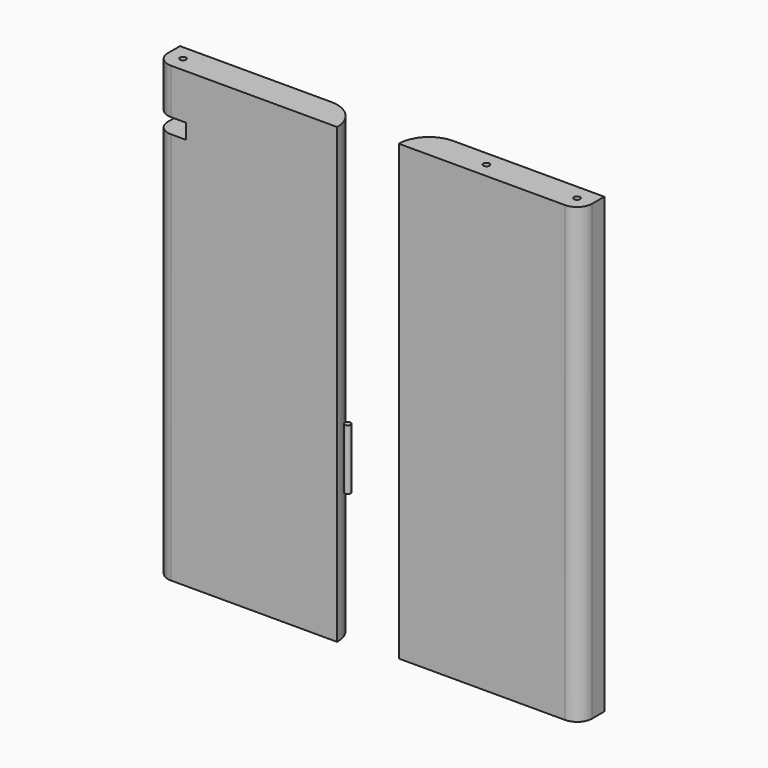
from build123d import *

# Parameters (mm, degrees)
F1_DEPTH  = 10
F0_W      = 60
F0_H      = 150
F2_R      = 5
F2_2_R    = 5
F4_R      = 9.99999
F4_2_R    = 9.99999
F3_W      = 30
F3_H      = 2
F5_DEPTH  = 8
F6_R      = 1
F7_DEPTH  = 20
F8_R      = 1
F9_DEPTH  = 10
F10_R     = 1
F11_DEPTH = 10
F12_R     = 1
F13_DEPTH = 10
F14_R     = 1
F15_DEPTH = 10
F16_R     = 1
F17_DEPTH = 20


# Not quite as in the source:
# - a fillet or chamfer is up to 0.001 mm smaller than in the source, because OpenCascade refuses the exact size


with BuildPart() as f1:
    # F0 (on Front) → F1 (new body)
    with BuildSketch(Plane.XZ):
        Polygon((-17.6528605427, 79.6767238528), (-77.6528605427, 79.6767238528), (-77.6528605427, 64.6767238528), (-67.6528605427, 64.6767238528), (-67.6528605427, 59.6767238528), (-77.6528605427, 59.6767238528), (-77.6528605427, -70.3232761472), (-17.6528605427, -70.3232761472), align=None)
    extrude(amount=F1_DEPTH)

    # F2
    f2_edges = [f1.edges().sort_by_distance(p)[0] for p in [
        (-77.652861, -10, 72.176724),
        (-77.652861, -10, -5.323276),
    ]]
    fillet(f2_edges, radius=F2_R)

    # F4#2 (radius 10 in the source; OpenCascade refuses exactly that, so slightly less here)
    f4_2_edges = [f1.edges().sort_by_distance(p)[0] for p in [
        (-17.652861, 0, 4.676724),
    ]]
    fillet(f4_2_edges, radius=F4_2_R)

    # F8 (on face) → F9 (cut)
    with BuildSketch(Plane(origin=(0, 0, -70.3232761472), x_dir=(1, 0, 0), z_dir=(0, 0, -1))):
        with Locations((-72.6528605427, 5)):
            Circle(F8_R)
    extrude(amount=-F9_DEPTH, mode=Mode.SUBTRACT)

    # F12 (on face) → F13 (cut)
    with BuildSketch(Plane.XY.offset(79.6767238528)):
        with Locations((-72.6528605427, -5)):
            Circle(F12_R)
    extrude(amount=-F13_DEPTH, mode=Mode.SUBTRACT)


with BuildPart() as f1b:
    # F0 (on Front) → F1, piece 2 (new body)
    with BuildSketch(Plane.XZ):
        with Locations((32.7451354545, 6.4557090402)):
            Rectangle(F0_W, F0_H)
    extrude(amount=F1_DEPTH)

    # F2#2
    f2_2_edges = [f1b.edges().sort_by_distance(p)[0] for p in [
        (62.745135, -10, 6.455709),
    ]]
    fillet(f2_2_edges, radius=F2_2_R)

    # F4 (radius 10 in the source; OpenCascade refuses exactly that, so slightly less here)
    f4_edges = [f1b.edges().sort_by_distance(p)[0] for p in [
        (2.745135, 0, 6.455709),
    ]]
    fillet(f4_edges, radius=F4_R)

    # F3 (on face) → F5 (cut)
    with BuildSketch(Plane(origin=(0, 0, 0), x_dir=(-1, 0, 0), z_dir=(0, 1, 0))):
        with Locations((-27.7451354545, 67.4557090402)):
            Rectangle(F3_W, F3_H)
    extrude(amount=-F5_DEPTH, mode=Mode.SUBTRACT)

    # F6 (on face) → F7 (cut)
    with BuildSketch(Plane.XY.offset(81.4557090402)):
        with Locations((27.7451354545, -5)):
            Circle(F6_R)
    extrude(amount=-F7_DEPTH, mode=Mode.SUBTRACT)

    # F10 (on face) → F11 (cut)
    with BuildSketch(Plane(origin=(0, 0, -68.5442909598), x_dir=(1, 0, 0), z_dir=(0, 0, -1))):
        with Locations((57.7451354545, 5)):
            Circle(F10_R)
    extrude(amount=-F11_DEPTH, mode=Mode.SUBTRACT)

    # F14 (on face) → F15 (cut)
    with BuildSketch(Plane.XY.offset(81.4557090402)):
        with Locations((57.7451354545, -5)):
            Circle(F14_R)
    extrude(amount=-F15_DEPTH, mode=Mode.SUBTRACT)


with BuildPart() as f17:
    # F16 (on Top) → F17 (new body)
    with BuildSketch(Plane.XY):
        with Locations((16.5821891278, -48.4209731221)):
            Circle(F16_R)
    extrude(amount=F17_DEPTH)


solid = Compound([f1.part, f1b.part, f17.part])
